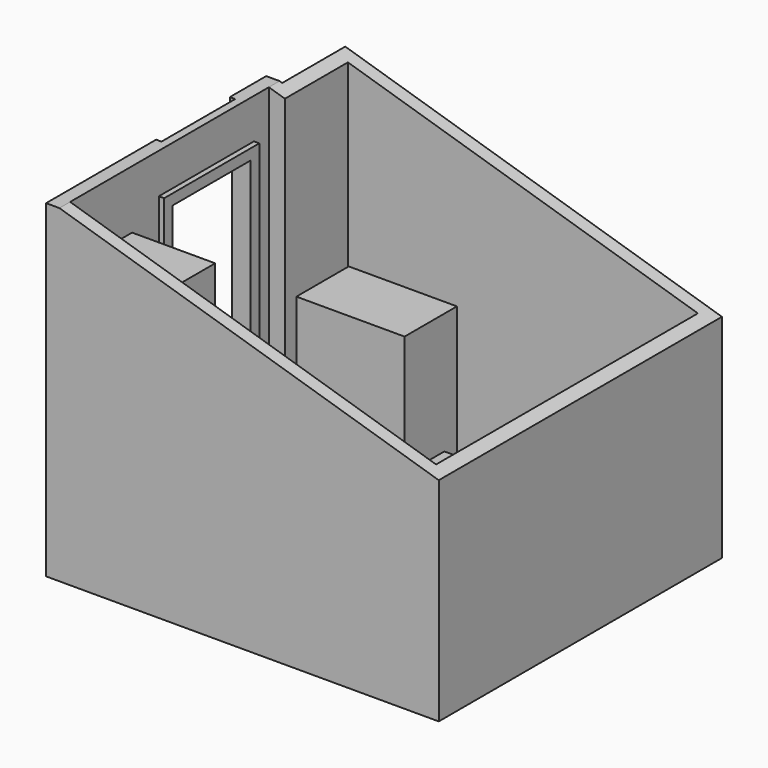
from build123d import *

# Parameters (mm, degrees)
F1_DEPTH      = 100
F2_DEPTH      = 2460
F0_W          = 85
F0_H          = 900
F3_DEPTH      = 720
F4_DEPTH      = 10
F6_DEPTH      = 1484.5868141508
F6_DEPTH_BACK = 1165.4151858492
F7_W          = 890
F7_H          = 300
F8_DEPTH      = 40
F9_W          = 730
F9_H          = 1980
F10_DEPTH     = 140.001
F12_W         = 810
F12_H         = 490
F13_DEPTH     = 1100
F12_W_2       = 1410
F12_H_2       = 1960
F14_DEPTH     = 400
F12_W_3       = 380
F12_H_3       = 400
F15_DEPTH     = 600
F17_DEPTH     = 580


with BuildPart() as f1:
    # F0 (on Top) → F1 (new body)
    with BuildSketch(Plane.XY):
        Polygon((1337.0921968033, 1384.5858141508), (-1282.9078031967, 1384.5858141508), (-1282.9078031967, 794.5858141508), (-1402.9078031967, 794.5858141508), (-1402.9078031967, 654.5858141508), (-1362.9078031967, 654.5858141508), (-1362.9078031967, -235.4141858492), (-1402.9078031967, -235.4141858492), (-1402.9078031967, -1065.4141858492), (1337.0921968033, -1065.4141858492), align=None)
        Polygon((-1377.9078031967, 769.5858141508), (-1257.9078031967, 769.5858141508), (-1257.9078031967, 1359.5858141508), (1312.0921968033, 1359.5858141508), (1312.0921968033, 534.5858141508), (1312.0921968033, -365.4141858492), (1312.0921968033, -1040.4141858492), (-1377.9078031967, -1040.4141858492), (-1377.9078031967, -260.4141858492), (-1337.9078031967, -260.4141858492), (-1337.9078031967, 679.5858141508), (-1377.9078031967, 679.5858141508), align=None, mode=Mode.SUBTRACT)
    extrude(amount=F1_DEPTH)

    # F0 (on Top) → F2 (join)
    with BuildSketch(Plane.XY):
        Polygon((-1502.9078031967, -135.4141858492), (-1502.9078031967, -1165.4141858492), (1437.0921968033, -1165.4141858492), (1437.0921968033, 1484.5858141508), (-1382.9078031967, 1484.5858141508), (-1382.9078031967, 894.5858141508), (-1502.9078031967, 894.5858141508), (-1502.9078031967, 554.5858141508), (-1462.9078031967, 554.5858141508), (-1462.9078031967, -135.4141858492), align=None)
        Polygon((-1282.9078031967, 794.5858141508), (-1282.9078031967, 1384.5858141508), (1337.0921968033, 1384.5858141508), (1337.0921968033, -1065.4141858492), (-1402.9078031967, -1065.4141858492), (-1402.9078031967, -235.4141858492), (-1362.9078031967, -235.4141858492), (-1362.9078031967, 654.5858141508), (-1402.9078031967, 654.5858141508), (-1402.9078031967, 794.5858141508), align=None, mode=Mode.SUBTRACT)
    extrude(amount=F2_DEPTH)

    # F0 (on Top) → F3 (join)
    with BuildSketch(Plane.XY):
        with Locations((1269.5921968033, 84.5858141508)):
            Rectangle(F0_W, F0_H)
    extrude(amount=F3_DEPTH)

    # F5 (on Front) → F6 (cut, two sides)
    with BuildSketch(Plane.XZ) as f6_sk:
        Polygon((1437.0921968033, 2460), (-1402.9078031967, 2460), (1437.0921968033, 1590), align=None)
    extrude(amount=-F6_DEPTH, mode=Mode.SUBTRACT)
    extrude(f6_sk.sketch, amount=F6_DEPTH_BACK, mode=Mode.SUBTRACT)

    # F7 (on face) → F8 (cut, through all)
    with BuildSketch(Plane.YZ.offset(-1362.9078031967)):
        with Locations((209.5858141508, 2310)):
            Rectangle(F7_W, F7_H)
    extrude(amount=-F8_DEPTH, mode=Mode.SUBTRACT)

    # F9 (on face) → F10 (cut, through all)
    with BuildSketch(Plane.YZ.offset(-1362.9078031967)):
        with Locations((209.5858141508, 1090)):
            Rectangle(F9_W, F9_H)
    extrude(amount=-F10_DEPTH, mode=Mode.SUBTRACT)


with BuildPart() as f4:
    # F0 (on Top) → F4 (new body)
    with BuildSketch(Plane.XY):
        Polygon((-1257.9078031967, 1359.5858141508), (-1257.9078031967, 769.5858141508), (-1377.9078031967, 769.5858141508), (-1377.9078031967, 679.5858141508), (-1337.9078031967, 679.5858141508), (-1337.9078031967, -260.4141858492), (-1377.9078031967, -260.4141858492), (-1377.9078031967, -1040.4141858492), (1312.0921968033, -1040.4141858492), (1312.0921968033, -365.4141858492), (1227.0921968033, -365.4141858492), (1227.0921968033, 534.5858141508), (1312.0921968033, 534.5858141508), (1312.0921968033, 1359.5858141508), align=None)
    extrude(amount=-F4_DEPTH)


with BuildPart() as f13:
    # F12 (on face) → F13 (new body)
    with BuildSketch(Plane.XY):
        with Locations((-847.9078031967, 1109.5858141508)):
            Rectangle(F12_W, F12_H)
    extrude(amount=F13_DEPTH)


with BuildPart() as f14:
    # F12 (on face) → F14 (new body)
    with BuildSketch(Plane.XY):
        with Locations((512.0921968033, -55.4141858492)):
            Rectangle(F12_W_2, F12_H_2)
    extrude(amount=F14_DEPTH)


with BuildPart() as f15:
    # F12 (on face) → F15 (new body)
    with BuildSketch(Plane.XY):
        with Locations((-387.9078031967, -835.4141858492)):
            Rectangle(F12_W_3, F12_H_3)
    extrude(amount=F15_DEPTH)


with BuildPart() as f17:
    # F16 (on face) → F17 (new body)
    with BuildSketch(Plane(origin=(0, -1065.4141858492, 0), x_dir=(-1, 0, 0), z_dir=(0, 1, 0))):
        Polygon((802.9078031967, 2000), (1402.9078031967, 2000), (1402.9078031967, 2022), (780.9078031967, 2022), (780.9078031967, 0), (802.9078031967, 0), align=None)
    extrude(amount=F17_DEPTH)


solid = Compound([f1.part, f4.part, f13.part, f14.part, f15.part, f17.part])
